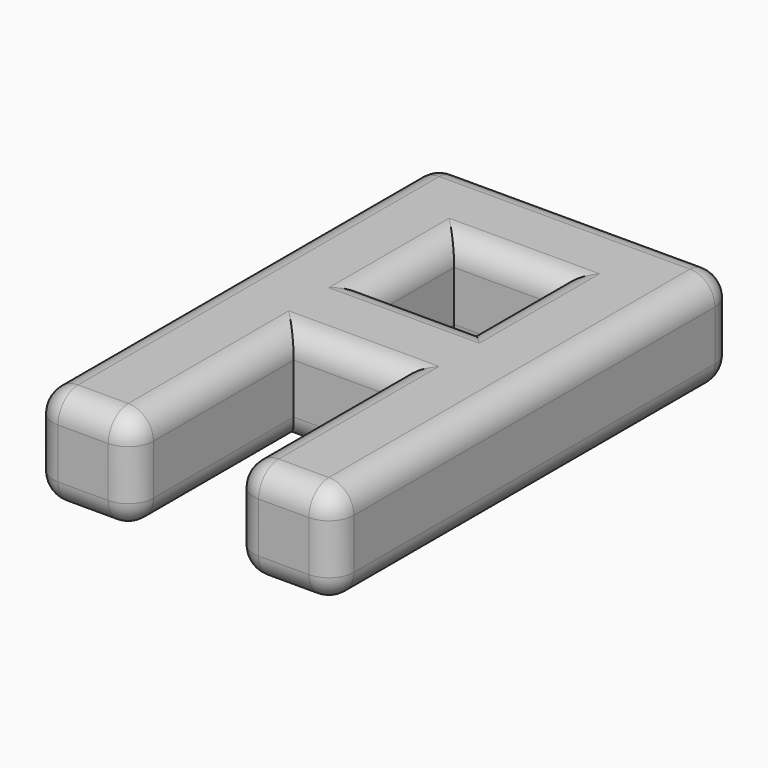
from build123d import *

# Parameters (mm, degrees)
F0_W     = 15.24
F0_H     = 25.4
F1_DEPTH = 5.08
F2_W     = 5.08
F2_H     = 5.08
F2_H_2   = 10.16
F3_DEPTH = 5.08
F4_R     = 1.27


with BuildPart() as f1:
    # F0 (on Top) → F1 (new body)
    with BuildSketch(Plane.XY):
        Rectangle(F0_W, F0_H)
    extrude(amount=F1_DEPTH)

    # F2 (on face) → F3 (cut)
    with BuildSketch(Plane.XY.offset(5.08)):
        with Locations((0, 5.08)):
            Rectangle(F2_W, F2_H)
        with Locations((0, -7.62)):
            Rectangle(F2_W, F2_H_2)
    extrude(amount=-F3_DEPTH, mode=Mode.SUBTRACT)

    # F4
    f4_edges = [f1.edges().sort_by_distance(p)[0] for p in [
        (-7.62, 12.7, 2.54),
        (-7.62, -12.7, 2.54),
        (0, 2.54, 5.08),
        (2.54, 5.08, 5.08),
        (-2.54, 5.08, 5.08),
        (0, 7.62, 5.08),
        (0, 12.7, 5.08),
        (0, 12.7, 0),
        (7.62, 12.7, 2.54),
        (0, -2.54, 5.08),
        (0, -2.54, 0),
        (2.54, -7.62, 5.08),
        (-2.54, -7.62, 5.08),
        (7.62, 0, 0),
        (7.62, 0, 5.08),
        (7.62, -12.7, 2.54),
        (5.08, -12.7, 5.08),
        (5.08, -12.7, 0),
        (2.54, -12.7, 2.54),
        (-5.08, -12.7, 5.08),
        (-2.54, -12.7, 2.54),
        (-7.62, 0, 5.08),
        (-5.08, -12.7, 0),
        (0, 2.54, 0),
        (-2.54, 5.08, 0),
        (0, 7.62, 0),
        (2.54, 5.08, 0),
        (-7.62, 0, 0),
        (-2.54, -7.62, 0),
        (2.54, -7.62, 0),
    ]]
    fillet(f4_edges, radius=F4_R)


solid = f1.part
